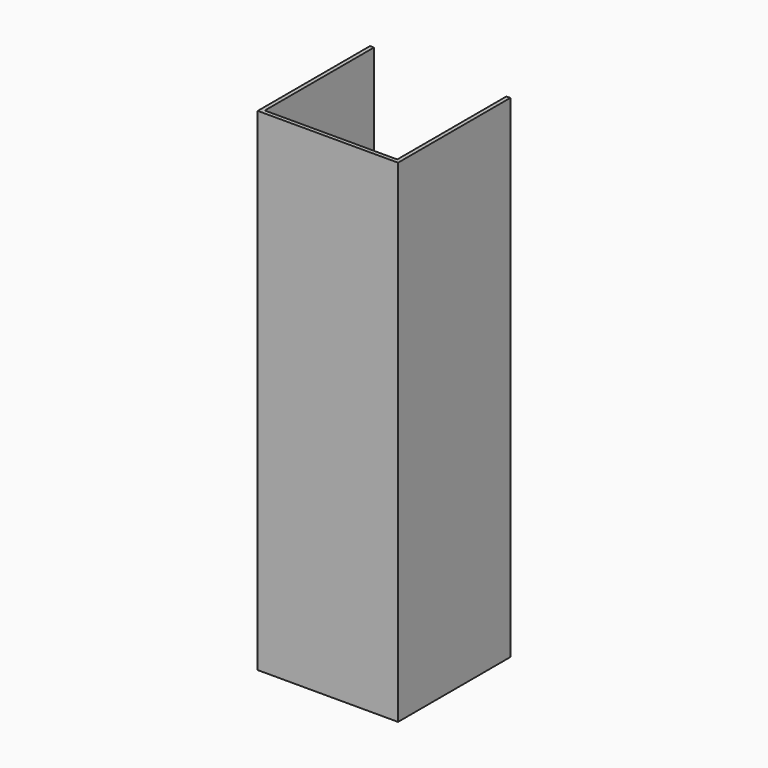
from build123d import *

# Parameters (mm, degrees)
F0_W     = 570
F0_H     = 570
F1_DEPTH = 2000
F2_T     = -16


# Not quite as in the source:
# - a feature names something its author has since deleted; it is built from what else it names


with BuildPart() as f1:
    # F0 (on Top) → F1 (new body)
    with BuildSketch(Plane.XY):
        with Locations((-285, -285)):
            Rectangle(F0_W, F0_H)
    extrude(amount=F1_DEPTH)

    # F2
    f2_openings = [f1.faces().sort_by_distance(p)[0] for p in [
        (-285, 0, 1000),
        (-285, -285, 2000),
        (-285, -285, 0),
    ]]
    offset(amount=F2_T, openings=f2_openings)


solid = f1.part
